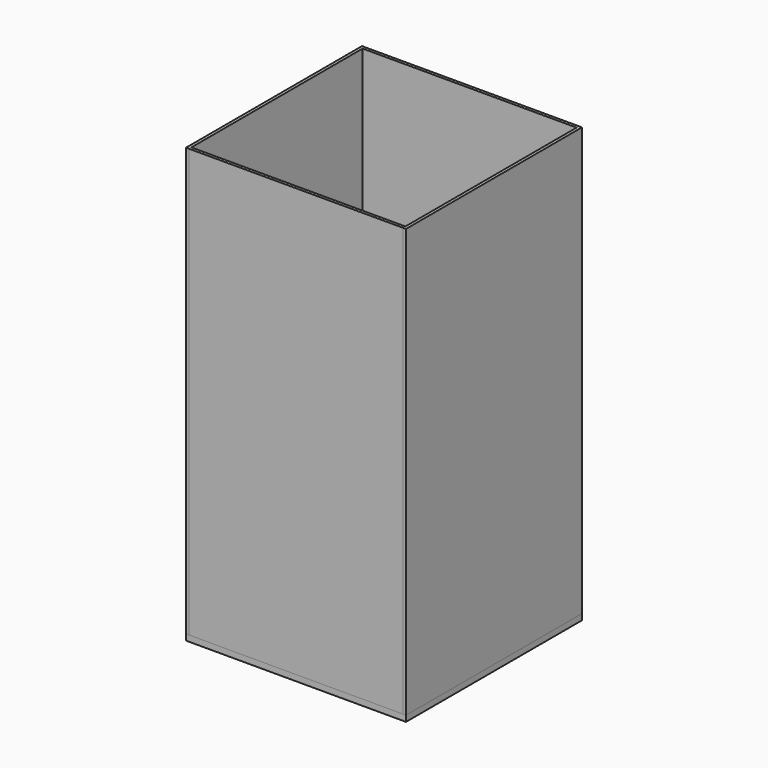
from build123d import *

# Parameters (mm, degrees)
F0_W     = 469.9
F0_H     = 469.9
F1_DEPTH = 12.7
F5_W     = 457.2
F5_H     = 6.35
F6_DEPTH = 914.4
F2_W     = 6.35
F2_H     = 469.9
F3_W     = 6.35
F3_H     = 469.9
F4_W     = 457.2
F4_H     = 6.35


# Not quite as in the source:
# - a length typed as a fraction of an inch, garbled in the dataset ("3 / 203.2 mm" for 3/8 in), is restored


with BuildPart() as f1:
    # F0 (on Top) → F1 (new body)
    with BuildSketch(Plane.XY):
        with Locations((234.95, 234.95)):
            Rectangle(F0_W, F0_H)
    extrude(amount=F1_DEPTH)


with BuildPart() as f6:
    # F5 (on face) → F6 (new body)
    with BuildSketch(Plane.XY.offset(12.7)):
        with Locations((234.95, 3.175)):
            Rectangle(F5_W, F5_H)
    extrude(amount=F6_DEPTH)


with BuildPart() as f6b:
    # F2 (on face) → F6, piece 2 (new body)
    with BuildSketch(Plane.XY.offset(12.7)):
        with Locations((3.175, 234.95)):
            Rectangle(F2_W, F2_H)
    extrude(amount=F6_DEPTH)


with BuildPart() as f6c:
    # F3 (on face) → F6, piece 3 (new body)
    with BuildSketch(Plane.XY.offset(12.7)):
        with Locations((466.725, 234.95)):
            Rectangle(F3_W, F3_H)
    extrude(amount=F6_DEPTH)


with BuildPart() as f6d:
    # F4 (on face) → F6, piece 4 (new body)
    with BuildSketch(Plane.XY.offset(12.7)):
        with Locations((234.95, 466.725)):
            Rectangle(F4_W, F4_H)
    extrude(amount=F6_DEPTH)


solid = Compound([f1.part, f6.part, f6b.part, f6c.part, f6d.part])
